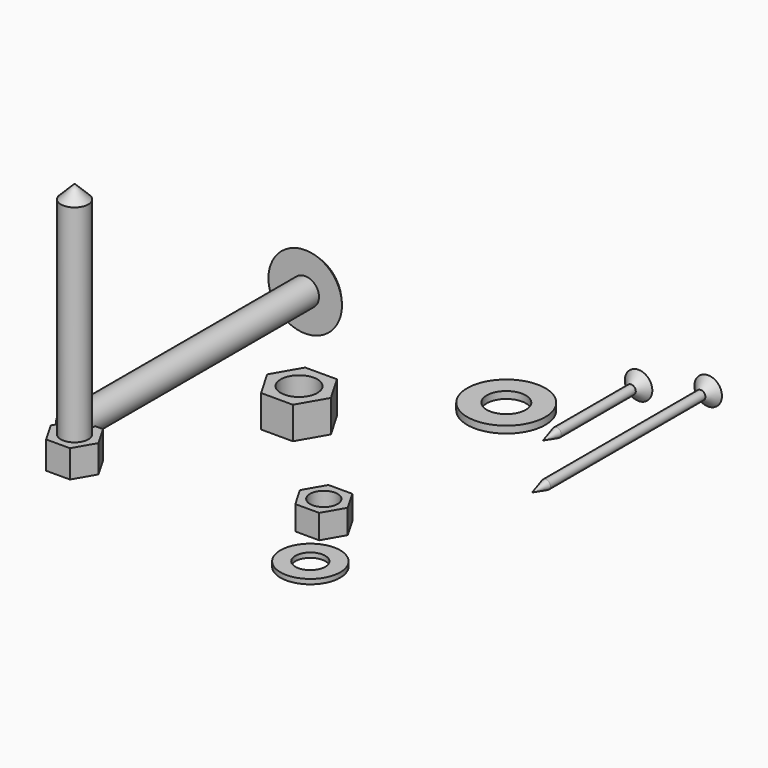
from build123d import *

# Parameters (mm, degrees)
F0_R      = 6.35
F1_DEPTH  = 11.1125
F2_R      = 13.49375
F2_R_2    = 6.746875
F3_DEPTH  = 2.413
F6_R      = 4.7625
F7_DEPTH  = 8.334375
F8_R      = 10.31875
F8_R_2    = 5.159375
F9_DEPTH  = 1.651
F14_DEPTH = 9.525
F15_DEPTH = 76.2
F16_SIZE  = 4.7625


# Not quite as in the source:
# - a length typed as a fraction of an inch, garbled in the dataset ("3 / 203.2 mm" for 3/8 in), is restored


with BuildPart() as f1:
    # F0 (on Top) → F1 (new body)
    with BuildSketch(Plane.XY):
        Polygon((5.499261314, 9.525), (-5.499261314, 9.525), (-10.9985226281, 0), (-5.499261314, -9.525), (5.499261314, -9.525), (10.9985226281, 0), align=None)
        Circle(F0_R, mode=Mode.SUBTRACT)
    extrude(amount=F1_DEPTH)


with BuildPart() as f3:
    # F2 (on Top) → F3 (new body)
    with BuildSketch(Plane.XY):
        with Locations((39.2041653395, 40.4630117118)):
            Circle(F2_R)
        with Locations((39.2041653395, 40.4630117118)):
            Circle(F2_R_2, mode=Mode.SUBTRACT)
    extrude(amount=F3_DEPTH)


with BuildPart() as f5:
    # F4 (on Top) → F5 (revolve)
    with BuildSketch(Plane.XY):
        with BuildLine():
            Line((-46.4556922868, -40.868859118), (-46.4556922868, 60.731140882))
            Line((-46.4556922868, 60.731140882), (-46.4556922868, 67.081140882))
            ThreePointArc((-46.4556922868, 67.081140882), (-53.5552081154, 65.4051725392), (-59.1556922868, 60.731140882))
            Line((-59.1556922868, 60.731140882), (-51.2181922868, 60.731140882))
            Line((-51.2181922868, 60.731140882), (-51.2181922868, -40.868859118))
            Line((-51.2181922868, -40.868859118), (-46.4556922868, -40.868859118))
        make_face()
    revolve(axis=Axis((-46.4556922868, 9.931140882, 0), (0, -1, 0)))


with BuildPart() as f7:
    # F6 (on Top) → F7 (new body)
    with BuildSketch(Plane.XY):
        Polygon((47.1631364482, -35.9566703924), (38.9142444772, -35.9566703924), (34.7897984917, -43.1004203924), (38.9142444772, -50.2441703924), (47.1631364482, -50.2441703924), (51.2875824338, -43.1004203924), align=None)
        with Locations((43.0386904627, -43.1004203924)):
            Circle(F6_R, mode=Mode.SUBTRACT)
    extrude(amount=F7_DEPTH)


with BuildPart() as f9:
    # F8 (on Top) → F9 (new body)
    with BuildSketch(Plane.XY):
        with Locations((54.9289397895, -63.7831166387)):
            Circle(F8_R)
        with Locations((54.9289397895, -63.7831166387)):
            Circle(F8_R_2, mode=Mode.SUBTRACT)
    extrude(amount=F9_DEPTH)


with BuildPart() as f11:
    # F10 (on Top) → F11 (revolve)
    with BuildSketch(Plane.XY):
        Polygon((57.8924338935, 74.1986898454), (53.1299338935, 74.1986898454), (56.3049338935, 71.0236898454), (56.3049338935, 38.8483205024), (57.8924338935, 32.9236898454), align=None)
    revolve(axis=Axis((57.8924338935, 53.5611898454, 0), (0, -1, 0)))


with BuildPart() as f13:
    # F12 (on Top) → F13 (revolve)
    with BuildSketch(Plane.XY):
        Polygon((74.5598336721, 83.4161932281), (69.7973336721, 83.4161932281), (72.9723336721, 80.2411932281), (72.9723336721, 13.3236167875), (74.5598336721, 7.3989861305), align=None)
    revolve(axis=Axis((74.5598336721, 45.4075896793, 0), (0, -1, 0)))


with BuildPart() as f14:
    # F6 (on Top) → F14 (new body)
    with BuildSketch(Plane.XY):
        Polygon((-34.7897984917, -43.1004203924), (-38.9142444772, -35.9566703924), (-47.1631364482, -35.9566703924), (-51.2875824338, -43.1004203924), (-47.1631364482, -50.2441703924), (-38.9142444772, -50.2441703924), align=None)
        with Locations((-43.0386904627, -43.1004203924)):
            Circle(F6_R, mode=Mode.SUBTRACT)
        with Locations((-43.0386904627, -43.1004203924)):
            Circle(F6_R)
    extrude(amount=-F14_DEPTH)

    # F6 (on Top) → F15 (join)
    with BuildSketch(Plane.XY):
        with Locations((-43.0386904627, -43.1004203924)):
            Circle(F6_R)
    extrude(amount=F15_DEPTH)

    # F16
    f16_edges = [f14.edges().sort_by_distance(p)[0] for p in [
        (-47.80119, -43.10042, 76.2),
    ]]
    chamfer(f16_edges, length=F16_SIZE)


solid = Compound([f1.part, f3.part, f5.part, f7.part, f9.part, f11.part, f13.part, f14.part])
